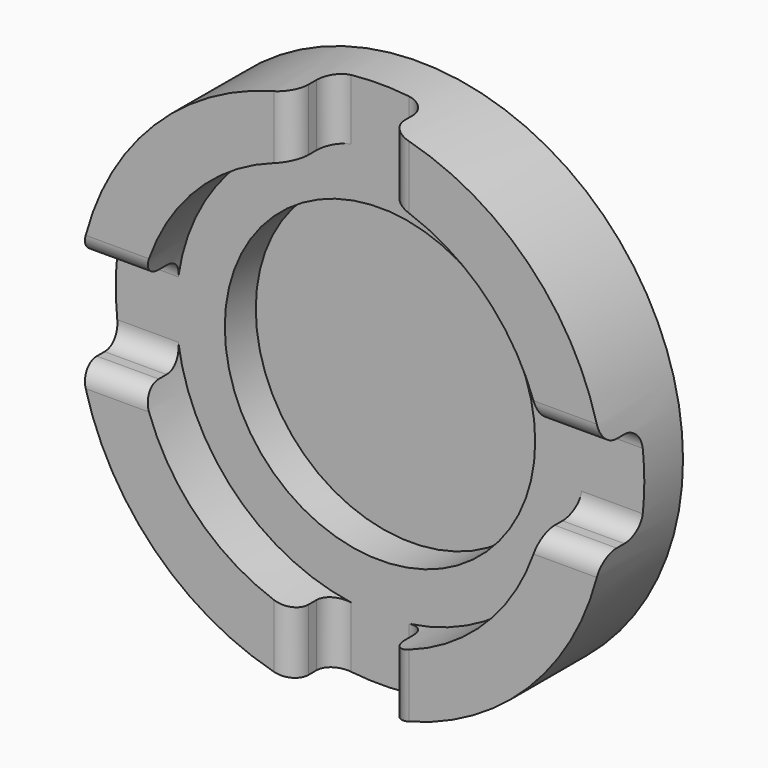
from build123d import *

# Parameters (mm, degrees)
F0_R            = 40.7218115667
F1_DEPTH        = 2.54
F0_R_2          = 53.4529743156
F2_DEPTH        = 12.7
F0_R_3          = 69.3420856698
F3_DEPTH        = 25.4
F4_W            = 23.4954506159
F4_H            = 25.2576172352
F5_DEPTH        = 12.7
F5_COPIES_COUNT = 4
F6_R            = 5.08


# Not quite as in the source:
# - a pattern or mirror of a feature is missing from the dataset's text; its kind, count and spacing are read off the source's solid


with BuildPart() as f1:
    # F0 (on Front) → F1 (new body)
    with BuildSketch(Plane.XZ):
        Circle(F0_R)
    extrude(amount=F1_DEPTH)


with BuildPart() as f2:
    # F0 (on Front) → F2 (new body)
    with BuildSketch(Plane.XZ):
        Circle(F0_R_2)
        Circle(F0_R, mode=Mode.SUBTRACT)
    extrude(amount=F2_DEPTH)

    # F0 (on Front) → F3 (join)
    with BuildSketch(Plane.XZ):
        Circle(F0_R_3)
        Circle(F0_R_2, mode=Mode.SUBTRACT)
    extrude(amount=F3_DEPTH)

    # F4 (on face) → F5 (cut)
    with BuildSketch(Plane.XZ.offset(25.4)):
        with Locations((-62.8503486514, 0)):
            Rectangle(F4_W, F4_H)
    f5 = extrude(amount=-F5_DEPTH, mode=Mode.SUBTRACT)

    # F5_copies: F5 ×4 about axis
    f5_copies_axis = Axis((0, 0, 0), (0, 1, 0))
    for i in range(1, F5_COPIES_COUNT):
        add(f5.rotate(f5_copies_axis, i * 360 / F5_COPIES_COUNT), mode=Mode.SUBTRACT)

    # F6
    f6_edges = [f2.edges().sort_by_distance(p)[0] for p in [
        (-60.06105, -12.7, 12.628809),
        (-60.06105, -12.7, -12.628809),
        (-60.06105, -25.4, -12.628809),
        (-60.06105, -25.4, 12.628809),
        (-12.628809, -12.7, -60.06105),
        (12.628809, -12.7, -60.06105),
        (60.06105, -12.7, -12.628809),
        (60.06105, -12.7, 12.628809),
        (12.628809, -12.7, 60.06105),
        (-12.628809, -12.7, 60.06105),
        (-12.628809, -25.4, 60.06105),
        (12.628809, -25.4, 60.06105),
        (60.06105, -25.4, 12.628809),
        (60.06105, -25.4, -12.628809),
        (12.628809, -25.4, -60.06105),
        (-12.628809, -25.4, -60.06105),
    ]]
    fillet(f6_edges, radius=F6_R)


solid = Compound([f1.part, f2.part])
